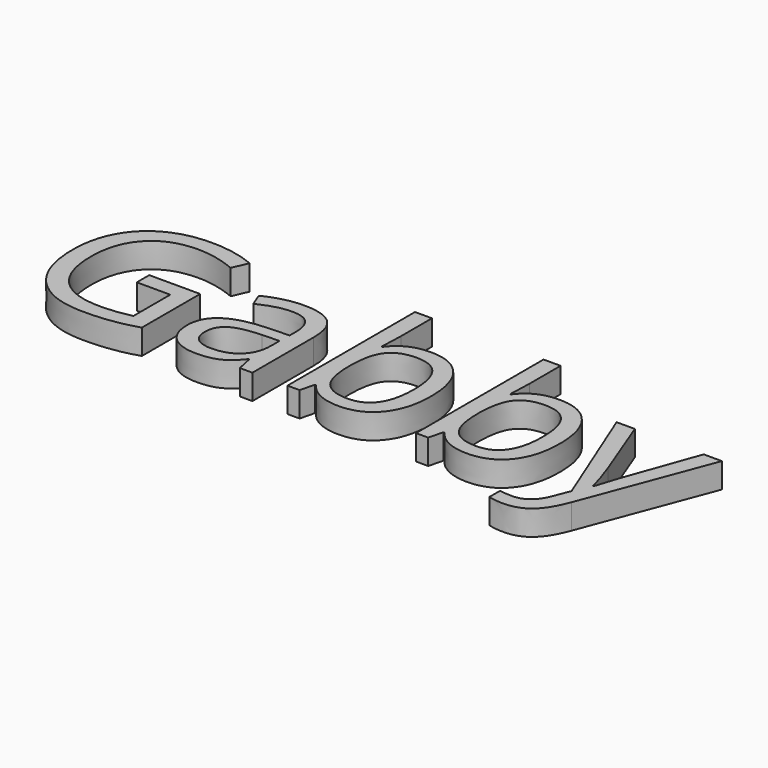
from build123d import *

# Parameters (mm, degrees)
F0_TEXT_SIZE = 53.2335317176
F1_DEPTH     = 6.35


# Not quite as in the source:
# - Text() gives the source's letters only with a copy of the font that has no kerning and outlines rounded to 1/6400 em; it was checked with that copy


with BuildPart() as f1:
    # F0 (on Top) → F1 (new body)
    with BuildSketch(Plane.XY):
        with Locations((-29.8240873963, -18.2058680803)):
            Text('Gabby', F0_TEXT_SIZE, font='Open Sans', text_align=(TextAlign.LEFT, TextAlign.BOTTOM))
    extrude(amount=F1_DEPTH)


solid = f1.part
